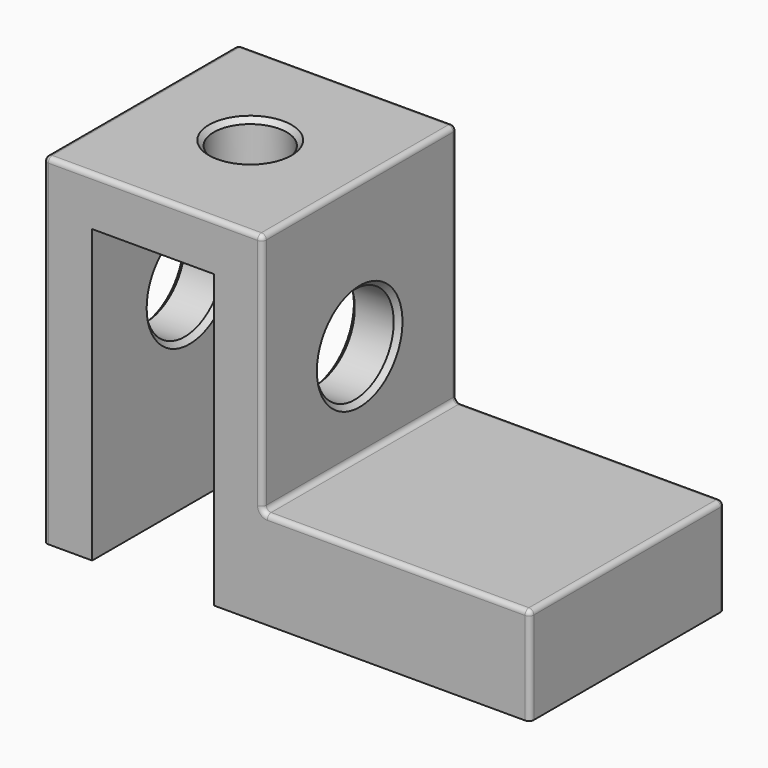
from build123d import *

# Parameters (mm, degrees)
F0_W     = 100
F0_H     = 50
F1_DEPTH = 20
F2_W     = 45
F2_H     = 50
F3_DEPTH = 50
F4_W     = 25
F4_H     = 60
F5_DEPTH = 50.001
F6_R     = 10
F7_DEPTH = 45
F8_R     = 7.5
F9_DEPTH = 10
F10_R    = 1
F11_SIZE = 1


with BuildPart() as f1:
    # F0 (on Top) → F1 (new body)
    with BuildSketch(Plane.XY):
        with Locations((50, 25)):
            Rectangle(F0_W, F0_H)
    extrude(amount=F1_DEPTH)

    # F2 (on face) → F3 (join)
    with BuildSketch(Plane.XY.offset(20)):
        with Locations((22.5, 25)):
            Rectangle(F2_W, F2_H)
    extrude(amount=F3_DEPTH)

    # F4 (on face) → F5 (cut, through all)
    with BuildSketch(Plane.XZ):
        with Locations((22.5, 30)):
            Rectangle(F4_W, F4_H)
    extrude(amount=-F5_DEPTH, mode=Mode.SUBTRACT)

    # F6 (on face) → F7 (cut, through all)
    with BuildSketch(Plane(origin=(0, 0, 0), x_dir=(0, -1, 0), z_dir=(-1, 0, 0))):
        with Locations((-25, 40)):
            Circle(F6_R)
    extrude(amount=-F7_DEPTH, mode=Mode.SUBTRACT)

    # F8 (on face) → F9 (cut, through all)
    with BuildSketch(Plane.XY.offset(70)):
        with Locations((22.5, 25)):
            Circle(F8_R)
    extrude(amount=-F9_DEPTH, mode=Mode.SUBTRACT)

    # F10
    f10_edges = [f1.edges().sort_by_distance(p)[0] for p in [
        (45, 25, 70),
        (45, 25, 20),
        (45, 0, 45),
        (22.5, 0, 70),
        (0, 0, 35),
        (0, 25, 70),
        (22.5, 50, 70),
        (45, 50, 45),
        (72.5, 50, 20),
        (100, 25, 20),
        (0, 50, 35),
        (100, 0, 10),
        (100, 50, 10),
        (72.5, 0, 20),
    ]]
    fillet(f10_edges, radius=F10_R)

    # F11
    f11_edges = [f1.edges().sort_by_distance(p)[0] for p in [
        (45, 35, 40),
        (10, 35, 40),
        (35, 35, 40),
        (0, 35, 40),
        (15, 25, 70),
        (15, 25, 60),
    ]]
    chamfer(f11_edges, length=F11_SIZE)


solid = f1.part
